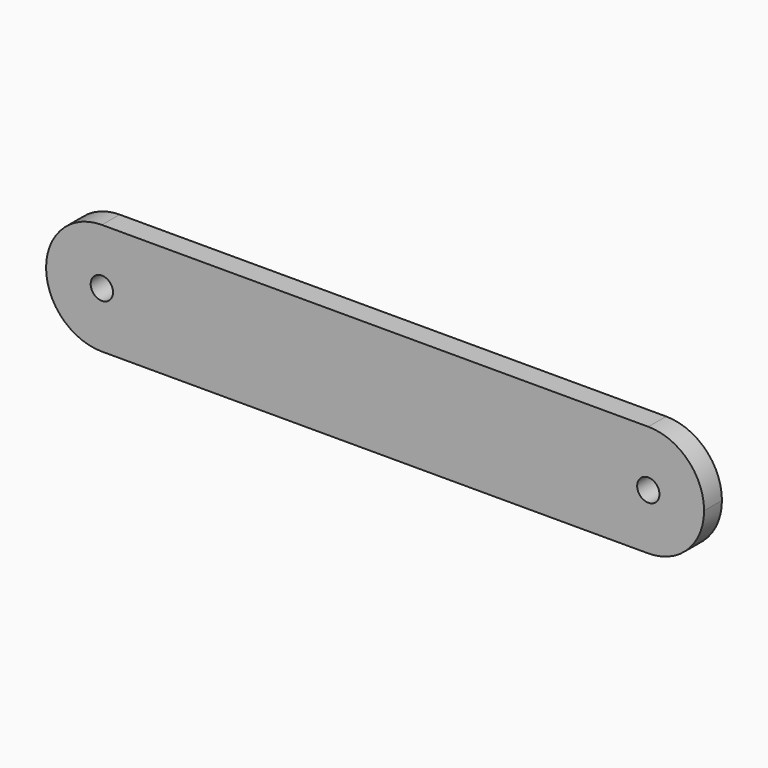
from build123d import *

# Parameters (mm, degrees)
F0_W     = 59
F0_H     = 10
F0_R     = 1
F1_DEPTH = 2
F2_R     = 4.99999


# Not quite as in the source:
# - a fillet or chamfer is up to 0.001 mm smaller than in the source, because OpenCascade refuses the exact size


with BuildPart() as f1:
    # F0 (on Front) → F1 (new body)
    with BuildSketch(Plane.XZ):
        with Locations((29.5, -5)):
            Rectangle(F0_W, F0_H)
        with Locations((5, -5)):
            Circle(F0_R, mode=Mode.SUBTRACT)
        with Locations((54, -5)):
            Circle(F0_R, mode=Mode.SUBTRACT)
    extrude(amount=F1_DEPTH)

    # F2 (radius 5 in the source; OpenCascade refuses exactly that, so slightly less here)
    f2_edges = [f1.edges().sort_by_distance(p)[0] for p in [
        (0, -1, 0),
        (0, -1, -10),
        (59, -1, -10),
        (59, -1, 0),
    ]]
    fillet(f2_edges, radius=F2_R)


solid = f1.part
